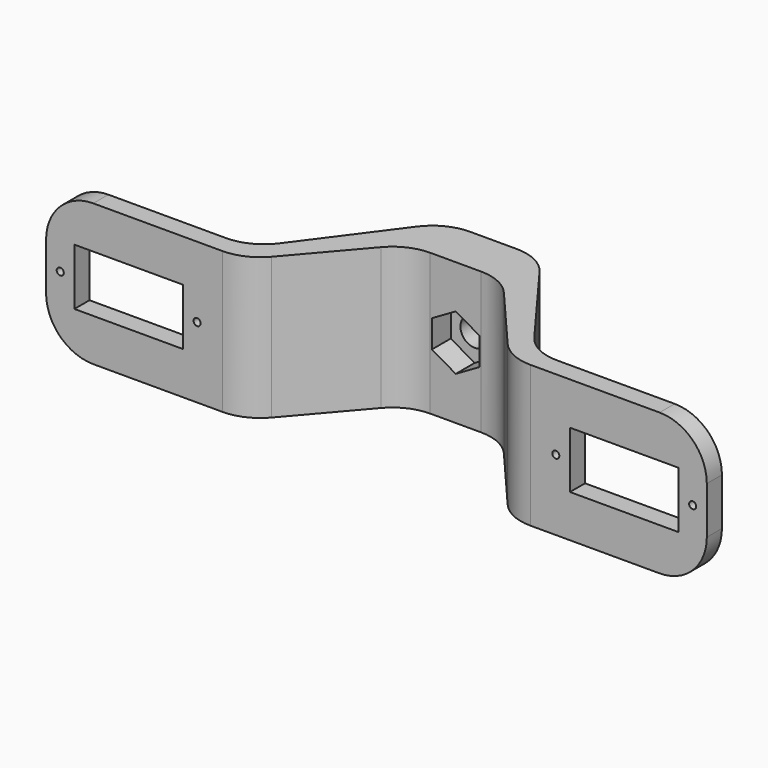
from build123d import *

# Parameters (mm, degrees)
F1_DEPTH = 30
F2_W     = 23
F2_H     = 12
F2_R     = 0.75
F3_DEPTH = 25
F4_R     = 10
F5_R     = 3
F6_DEPTH = 25
F7_DEPTH = 5


# Not quite as in the source:
# - a feature names something its author has since deleted; it is built from what else it names


with BuildPart() as f1:
    # F0 (on Top) → F1 (new body)
    with BuildSketch(Plane.XY):
        Polygon((30, 4), (10, 31), (-10, 31), (-30, 4), (-70, 4), (-70, 0), (-28, 0), (-10, 21), (10, 21), (28, 0), (70, 0), (70, 4), align=None)
    extrude(amount=F1_DEPTH)

    # F2 (on face) → F3 (cut)
    with BuildSketch(Plane(origin=(0, 4, 0), x_dir=(-1, 0, 0), z_dir=(0, 1, 0))):
        with Locations((52.5, 15)):
            Rectangle(F2_W, F2_H)
        with Locations((-52.5, 15)):
            Rectangle(F2_W, F2_H)
        with Locations((-38, 15)):
            Circle(F2_R)
        with Locations((-67, 15)):
            Circle(F2_R)
        with Locations((38, 15)):
            Circle(F2_R)
        with Locations((67, 15)):
            Circle(F2_R)
    extrude(amount=-F3_DEPTH, mode=Mode.SUBTRACT)

    # F4
    f4_edges = [f1.edges().sort_by_distance(p)[0] for p in [
        (-70, 2, 30),
        (-70, 2, 0),
        (70, 2, 30),
        (70, 2, 0),
        (30, 4, 15),
        (-30, 4, 15),
        (-10, 31, 15),
        (10, 31, 15),
        (-28, 0, 15),
        (-10, 21, 15),
        (10, 21, 15),
        (28, 0, 15),
    ]]
    fillet(f4_edges, radius=F4_R)

    # F5 (on face) → F6 (cut)
    with BuildSketch(Plane.XZ.offset(-21)):
        with Locations((0, 15)):
            Circle(F5_R)
    extrude(amount=-F6_DEPTH, mode=Mode.SUBTRACT)

    # F5 (on face) → F7 (cut)
    with BuildSketch(Plane.XZ.offset(-21)):
        Polygon((0, 9.1687622812), (5.05, 12.0843811406), (5.05, 17.9156188594), (0, 20.8312377188), (-5.05, 17.9156188594), (-5.05, 12.0843811406), align=None)
        with Locations((0, 15)):
            Circle(F5_R, mode=Mode.SUBTRACT)
    extrude(amount=-F7_DEPTH, mode=Mode.SUBTRACT)


solid = f1.part
